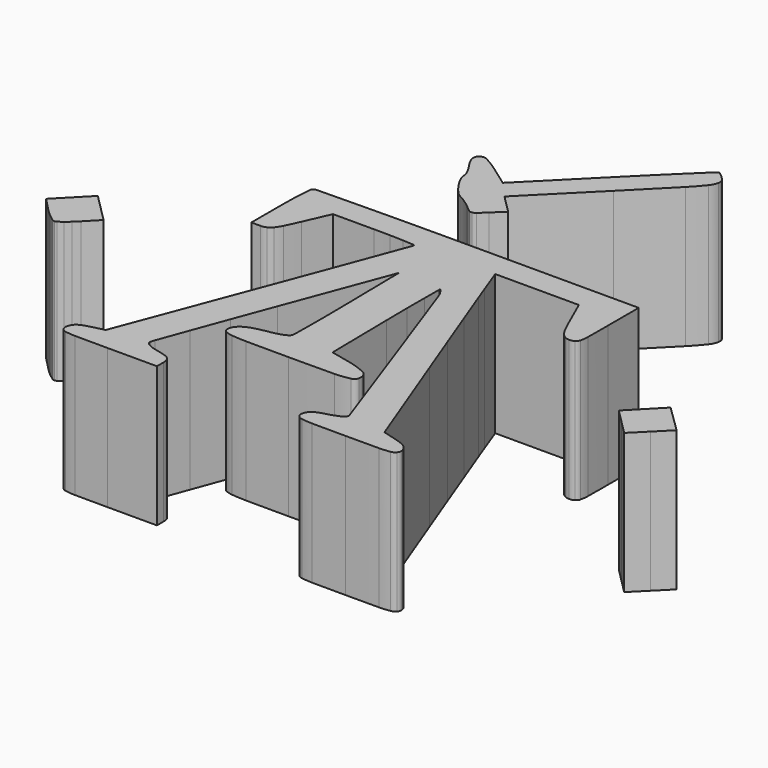
from build123d import *

# Parameters (mm, degrees)
F1_DEPTH = 25.4


# Not quite as in the source:
# - ends of sketch curves that miss each other by under 0.0002 mm in the source are joined


with BuildPart() as f1:
    # F0 (on Top) → F1 (new body)
    with BuildSketch(Plane.XY):
        with BuildLine():
            ThreePointArc((5.3278445908, 41.3714779095), (3.2465711293, 39.3070308207), (1.17245908, 37.2353889088))
            Line((1.17245908, 37.2353889088), (-9.5913702, 26.4470134))
            Line((-9.5913702, 26.4470134), (-12.7011938, 28.683204))
            ThreePointArc((-12.7011938, 28.683204), (-13.3183585785, 29.1173684963), (-13.9436757116, 29.5397069454))
            ThreePointArc((-13.9436757116, 29.5397069454), (-14.5193714679, 29.9086216736), (-15.1044112342, 30.2625312704))
            ThreePointArc((-15.1044112342, 30.2625312704), (-15.5950884738, 30.543091178), (-16.0913084379, 30.8137267723))
            ThreePointArc((-16.0913084379, 30.8137267723), (-16.2968587814, 30.8924942229), (-16.5153340201, 30.919394321))
            ThreePointArc((-16.5153340201, 30.919394321), (-16.9226686053, 30.8511854826), (-17.2859206172, 30.6546522226))
            ThreePointArc((-17.2859206172, 30.6546522226), (-17.5271690517, 30.364917692), (-17.6261968467, 30.0011334829))
            ThreePointArc((-17.6261968467, 30.0011334829), (-17.5891444827, 29.4731021199), (-17.4260613408, 28.9695197931))
            ThreePointArc((-17.4260613408, 28.9695197931), (-17.0829981706, 28.3120476284), (-16.6815115402, 27.6885323705))
            ThreePointArc((-16.6815115402, 27.6885323705), (-16.4130854245, 27.2958467266), (-16.1588952835, 26.8937997138))
            ThreePointArc((-16.1588952835, 26.8937997138), (-15.9263973461, 26.4923803768), (-15.7096472859, 26.082243352))
            ThreePointArc((-15.7096472859, 26.082243352), (-15.538374955, 25.7240460963), (-15.3811153362, 25.3594795088))
            ThreePointArc((-15.3811153362, 25.3594795088), (-15.3099545264, 25.1326203534), (-15.2773641169, 24.897105361))
            ThreePointArc((-15.2773641169, 24.897105361), (-15.1698479238, 24.2112132717), (-14.92665216, 23.5609324883))
            ThreePointArc((-14.92665216, 23.5609324883), (-14.4483979208, 22.6732535733), (-13.9104887011, 21.8204027876))
            ThreePointArc((-13.9104887011, 21.8204027876), (-13.3092790301, 21.0009126467), (-12.653090095, 20.2247464701))
            ThreePointArc((-12.653090095, 20.2247464701), (-12.116780938, 19.733761433), (-11.5001439659, 19.348471486))
            ThreePointArc((-11.5001439659, 19.348471486), (-11.1754765193, 19.1754158775), (-10.8590257516, 18.9877568523))
            ThreePointArc((-10.8590257516, 18.9877568523), (-10.478367161, 18.7427644682), (-10.1037639509, 18.488609845))
            ThreePointArc((-10.1037639509, 18.488609845), (-9.728007842, 18.2191836028), (-9.3588458321, 17.9407910626))
            ThreePointArc((-9.3588458321, 17.9407910626), (-9.0475467696, 17.6897316237), (-8.7459153929, 17.4271352824))
            ThreePointArc((-8.7459153929, 17.4271352824), (-8.3257547456, 17.0725057087), (-7.882386554, 16.7473563241))
            ThreePointArc((-7.882386554, 16.7473563241), (-7.6169836921, 16.6362047182), (-7.3292467909, 16.6373584517))
            ThreePointArc((-7.3292467909, 16.6373584517), (-7.0071387172, 16.7492612965), (-6.723922607, 16.9391689223))
            ThreePointArc((-6.723922607, 16.9391689223), (-6.0764353369, 17.5201639355), (-5.4415732409, 18.1149288306))
            Line((-5.4415732409, 18.1149288306), (-3.4675826, 20.0078086))
            Line((-3.4675826, 20.0078086), (-5.1281838, 21.6699084))
            Line((-5.1281838, 21.6699084), (-6.7888104, 23.3320082))
            Line((-6.7888104, 23.3320082), (4.1881806, 34.3331546))
            ThreePointArc((4.1881806, 34.3331546), (7.7930148251, 37.9604709487), (11.3897657807, 41.5958026114))
            ThreePointArc((11.3897657807, 41.5958026114), (12.523535317, 42.8119402167), (13.5904491586, 44.0871345239))
            ThreePointArc((13.5904491586, 44.0871345239), (14.0089149681, 44.7642866407), (14.2620308946, 45.518988275))
            ThreePointArc((14.2620308946, 45.518988275), (14.2451471296, 46.1366085958), (13.9493028376, 46.679031271))
            ThreePointArc((13.9493028376, 46.679031271), (13.705692071, 46.9401609641), (13.4545324122, 47.1940382124))
            ThreePointArc((13.4545324122, 47.1940382124), (13.2182987163, 47.4161332681), (12.9734957351, 47.6287454609))
            ThreePointArc((12.9734957351, 47.6287454609), (12.766987693, 47.794471902), (12.5548365797, 47.9529106388))
            ThreePointArc((12.5548365797, 47.9529106388), (12.4503936803, 48.0055735047), (12.3348495998, 48.0237798327))
            ThreePointArc((12.3348495998, 48.0237798327), (12.1880394684, 47.9952034702), (12.0624877712, 47.9139225334))
            ThreePointArc((12.0624877712, 47.9139225334), (10.4763017356, 46.3850143704), (8.8914892317, 44.8546824931))
            ThreePointArc((8.8914892317, 44.8546824931), (7.1047725577, 43.1180875785), (5.3278445908, 41.3714779095))
        make_face()
    extrude(amount=F1_DEPTH)


with BuildPart() as f1b:
    # F0 (on Top) → F1, piece 2 (new body)
    with BuildSketch(Plane.XY):
        with BuildLine():
            ThreePointArc((-28.9239708038, 8.2930357171), (-29.152995534, 8.2444468749), (-29.3471492398, 8.1136128535))
            ThreePointArc((-29.3471492398, 8.1136128535), (-29.4682601242, 7.9400663572), (-29.5223586626, 7.7354696381))
            ThreePointArc((-29.5223586626, 7.7354696381), (-29.5939202697, 6.8198574282), (-29.6566110746, 5.9035951827))
            ThreePointArc((-29.6566110746, 5.9035951827), (-29.7154841875, 4.8106745704), (-29.7535896341, 3.7168329073))
            ThreePointArc((-29.7535896341, 3.7168329073), (-29.7773750178, 2.4615506125), (-29.78531, 1.2060682))
            Line((-29.78531, 1.2060682), (-29.7853354, -5.26288))
            Line((-29.7853354, -5.26288), (-28.1046428, -5.26288))
            ThreePointArc((-28.1046428, -5.26288), (-27.6062777101, -5.2086551361), (-27.1310275761, -5.0491305899))
            ThreePointArc((-27.1310275761, -5.0491305899), (-26.7119543373, -4.7934727371), (-26.3618756212, -4.4493409597))
            ThreePointArc((-26.3618756212, -4.4493409597), (-25.9353004854, -3.8541164125), (-25.5779432646, -3.2149332556))
            ThreePointArc((-25.5779432646, -3.2149332556), (-24.973316268, -1.9417562352), (-24.391795328, -0.6578610928))
            Line((-24.391795328, -0.6578610928), (-22.3596454, 3.94716))
            Line((-22.3596454, 3.94716), (-14.8989034, 3.94716))
            ThreePointArc((-14.8989034, 3.94716), (-13.4684758142, 3.9410291097), (-12.0381522128, 3.922724452))
            ThreePointArc((-12.0381522128, 3.922724452), (-10.8336974413, 3.8935023943), (-9.6297757324, 3.8472710983))
            ThreePointArc((-9.6297757324, 3.8472710983), (-8.5991325983, 3.7981908828), (-7.5686922552, 3.7450220359))
            ThreePointArc((-7.5686922552, 3.7450220359), (-7.4759905736, 3.7020835845), (-7.4381868, 3.607181))
            ThreePointArc((-7.4381868, 3.607181), (-7.4503065364, 3.4718072468), (-7.4862802644, 3.3407392034))
            ThreePointArc((-7.4862802644, 3.3407392034), (-8.7724726688, -0.1083342689), (-10.0611279758, -3.5564882958))
            ThreePointArc((-10.0611279758, -3.5564882958), (-11.5008222297, -7.3994906511), (-12.9438803478, -11.2412311313))
            ThreePointArc((-12.9438803478, -11.2412311313), (-14.6549480198, -15.7720720161), (-16.3673799517, -20.3023974401))
            Line((-16.3673799517, -20.3023974401), (-25.2965712, -43.8719976))
            Line((-25.2965712, -43.8719976), (-27.7052786, -44.4677038))
            ThreePointArc((-27.7052786, -44.4677038), (-28.2874050524, -44.6307686568), (-28.8586889532, -44.8284949938))
            ThreePointArc((-28.8586889532, -44.8284949938), (-29.2562234773, -45.0160926822), (-29.6206904422, -45.261837527))
            ThreePointArc((-29.6206904422, -45.261837527), (-29.8817631628, -45.5163086696), (-30.0861395554, -45.8182124633))
            ThreePointArc((-30.0861395554, -45.8182124633), (-30.2370017448, -46.1704326022), (-30.323996421, -46.5435945421))
            ThreePointArc((-30.323996421, -46.5435945421), (-30.3007912145, -46.9830452901), (-30.1131180273, -47.3810805815))
            ThreePointArc((-30.1131180273, -47.3810805815), (-29.7883685131, -47.6800367128), (-29.375406369, -47.8359307716))
            ThreePointArc((-29.375406369, -47.8359307716), (-28.458843958, -47.95409568), (-27.5357843419, -47.99893212))
            ThreePointArc((-27.5357843419, -47.99893212), (-24.5755038228, -48.0175419738), (-21.6151714, -48.0237799114))
            Line((-21.6151714, -48.0237799114), (-12.6963424, -48.02378))
            Line((-12.6963424, -48.02378), (-12.6963424, -46.472602))
            ThreePointArc((-12.6963424, -46.472602), (-12.7302223523, -46.0551402422), (-12.8310496664, -45.6486211837))
            ThreePointArc((-12.8310496664, -45.6486211837), (-12.9862196969, -45.3438878864), (-13.2225719523, -45.0967576001))
            ThreePointArc((-13.2225719523, -45.0967576001), (-13.5940527082, -44.8590152554), (-14.0023554338, -44.6922515876))
            ThreePointArc((-14.0023554338, -44.6922515876), (-14.7423043874, -44.4823158012), (-15.4897324501, -44.3007988288))
            ThreePointArc((-15.4897324501, -44.3007988288), (-16.1129985159, -44.147980494), (-16.7292035242, -43.9688018542))
            ThreePointArc((-16.7292035242, -43.9688018542), (-17.1492723342, -43.808131553), (-17.5471652271, -43.5984765981))
            ThreePointArc((-17.5471652271, -43.5984765981), (-17.7890303402, -43.4148671659), (-17.9883130046, -43.1857457494))
            ThreePointArc((-17.9883130046, -43.1857457494), (-18.0830271411, -42.9662251402), (-18.0823332875, -42.7271440147))
            ThreePointArc((-18.0823332875, -42.7271440147), (-17.9922047416, -42.3644604005), (-17.8765595995, -42.0090894904))
            ThreePointArc((-17.8765595995, -42.0090894904), (-16.8761661379, -39.2778014924), (-15.8757102238, -36.5465363576))
            ThreePointArc((-15.8757102238, -36.5465363576), (-14.7208077115, -33.4124925221), (-13.561076035, -30.2802324757))
            ThreePointArc((-13.561076035, -30.2802324757), (-12.2081395128, -26.6521390034), (-10.8523743646, -23.025101585))
            Line((-10.8523743646, -23.025101585), (-3.823208, -4.27609))
            Line((-3.823208, -4.27609), (-3.6431474, -16.095472))
            ThreePointArc((-3.6431474, -16.095472), (-3.6136719859, -18.3874224076), (-3.5949994048, -20.6794862602))
            ThreePointArc((-3.5949994048, -20.6794862602), (-3.5906403215, -22.671554795), (-3.6006086996, -24.6636031458))
            ThreePointArc((-3.6006086996, -24.6636031458), (-3.617646112, -26.3742558468), (-3.6393185972, -28.0848561075))
            ThreePointArc((-3.6393185972, -28.0848561075), (-3.6695751202, -28.380444247), (-3.751135639, -28.6661654151))
            ThreePointArc((-3.751135639, -28.6661654151), (-3.8623048676, -28.8502564755), (-4.0302916076, -28.9845289711))
            ThreePointArc((-4.0302916076, -28.9845289711), (-4.3936920819, -29.1670538342), (-4.7676086151, -29.3269333921))
            ThreePointArc((-4.7676086151, -29.3269333921), (-5.2421745965, -29.4958060714), (-5.7260288389, -29.6358614262))
            ThreePointArc((-5.7260288389, -29.6358614262), (-6.2638999768, -29.7605658436), (-6.8069182424, -29.8605086892))
            ThreePointArc((-6.8069182424, -29.8605086892), (-8.0190343754, -30.0849752898), (-9.2190046989, -30.3672551586))
            ThreePointArc((-9.2190046989, -30.3672551586), (-10.0347957043, -30.6413342472), (-10.8059738626, -31.0233295773))
            ThreePointArc((-10.8059738626, -31.0233295773), (-11.3048691845, -31.3938263204), (-11.7115788922, -31.8636688024))
            ThreePointArc((-11.7115788922, -31.8636688024), (-11.9553040262, -32.3650301707), (-12.0390666, -32.9161648))
            ThreePointArc((-12.0390666, -32.9161648), (-11.9183040933, -33.3457718246), (-11.5913906605, -33.6495371718))
            ThreePointArc((-11.5913906605, -33.6495371718), (-10.9768409929, -33.8962944231), (-10.3275895017, -34.0268080175))
            ThreePointArc((-10.3275895017, -34.0268080175), (-8.956415452, -34.1382202475), (-7.5814175664, -34.1819462749))
            ThreePointArc((-7.5814175664, -34.1819462749), (-3.730521313, -34.202021893), (0.1204213997, -34.2087453118))
            ThreePointArc((0.1204213997, -34.2087453118), (4.2591148323, -34.1957032914), (8.3976463468, -34.1568489514))
            ThreePointArc((8.3976463468, -34.1568489514), (9.7846193058, -34.0684257366), (11.1554795133, -33.839822765))
            ThreePointArc((11.1554795133, -33.839822765), (11.6756540398, -33.5495614467), (11.9499271342, -33.0207901472))
            ThreePointArc((11.9499271342, -33.0207901472), (11.9492066699, -32.3183622866), (11.6908129953, -31.6651857299))
            ThreePointArc((11.6908129953, -31.6651857299), (11.5019501705, -31.4388791035), (11.2611464553, -31.268887852))
            ThreePointArc((11.2611464553, -31.268887852), (10.7620554787, -31.0215258697), (10.2523553101, -30.7968374028))
            ThreePointArc((10.2523553101, -30.7968374028), (9.6243180728, -30.5545425548), (8.9857341298, -30.3415904322))
            ThreePointArc((8.9857341298, -30.3415904322), (8.292834479, -30.1433250903), (7.5929489847, -29.9713396679))
            Line((7.5929489847, -29.9713396679), (4.0640254, -29.176345))
            Line((4.0640254, -29.176345), (3.8847522, -16.7660828))
            ThreePointArc((3.8847522, -16.7660828), (3.8551823479, -14.396553126), (3.8349222641, -12.0269255353))
            ThreePointArc((3.8349222641, -12.0269255353), (3.828650979, -10.0565823826), (3.835810793, -8.0862422521))
            ThreePointArc((3.835810793, -8.0862422521), (3.8489605343, -6.3857657005), (3.8644800933, -4.685309122))
            ThreePointArc((3.8644800933, -4.685309122), (3.9034557245, -4.6292112997), (3.9699407877, -4.644875361))
            ThreePointArc((3.9699407877, -4.644875361), (4.5804566767, -5.4623631608), (5.01846387, -6.3838644246))
            ThreePointArc((5.01846387, -6.3838644246), (8.2173339606, -15.3301399742), (11.410915362, -24.2783048372))
            ThreePointArc((11.410915362, -24.2783048372), (14.6850315999, -33.4763229), (17.9493538085, -42.6778213427))
            ThreePointArc((17.9493538085, -42.6778213427), (17.9716859269, -43.0784773813), (17.773638192, -43.4274853924))
            ThreePointArc((17.773638192, -43.4274853924), (17.6050453628, -43.5656397102), (17.4162550674, -43.6745783957))
            ThreePointArc((17.4162550674, -43.6745783957), (17.0602976651, -43.8353674885), (16.6993842935, -43.9847021908))
            ThreePointArc((16.6993842935, -43.9847021908), (16.2677640197, -44.1464384773), (15.8310367332, -44.2938283497))
            ThreePointArc((15.8310367332, -44.2938283497), (15.3719338033, -44.432389637), (14.9089588812, -44.5574051232))
            ThreePointArc((14.9089588812, -44.5574051232), (14.3669365543, -44.7146052049), (13.8365183342, -44.9073661764))
            ThreePointArc((13.8365183342, -44.9073661764), (13.4505758041, -45.0970991706), (13.0966666335, -45.3414319836))
            ThreePointArc((13.0966666335, -45.3414319836), (12.8387156081, -45.5939700437), (12.633215793, -45.8907599408))
            ThreePointArc((12.633215793, -45.8907599408), (12.4842625206, -46.2259033335), (12.3984867043, -46.5824838751))
            ThreePointArc((12.3984867043, -46.5824838751), (12.4272033206, -47.0131614318), (12.6302139233, -47.394073566))
            ThreePointArc((12.6302139233, -47.394073566), (12.9835009942, -47.6863609589), (13.4163811687, -47.8375498997))
            ThreePointArc((13.4163811687, -47.8375498997), (14.3847711602, -47.9542418982), (15.3591515091, -47.9987227082))
            ThreePointArc((15.3591515091, -47.9987227082), (18.4203719911, -48.0174952358), (21.4816436, -48.0237799213))
            ThreePointArc((21.4816436, -48.0237799213), (24.5291997473, -48.0174453865), (27.5767037643, -47.9985280802))
            ThreePointArc((27.5767037643, -47.9985280802), (28.5583528833, -47.9541157241), (29.5341071529, -47.8378721458))
            ThreePointArc((29.5341071529, -47.8378721458), (29.970152405, -47.6884335013), (30.3293647544, -47.3995887826))
            ThreePointArc((30.3293647544, -47.3995887826), (30.5350404946, -47.0255355391), (30.564807837, -46.5997040082))
            ThreePointArc((30.564807837, -46.5997040082), (30.4734690318, -46.2369946416), (30.3118540921, -45.8996783264))
            ThreePointArc((30.3118540921, -45.8996783264), (30.0828652781, -45.5927345053), (29.8010856701, -45.3334090197))
            ThreePointArc((29.8010856701, -45.3334090197), (29.4006427423, -45.0697274099), (28.9685803342, -44.8618681154))
            ThreePointArc((28.9685803342, -44.8618681154), (28.3527555007, -44.6348542972), (27.7256974666, -44.441018159))
            Line((27.7256974666, -44.441018159), (25.0966224, -43.7063896))
            Line((25.0966224, -43.7063896), (17.7223928, -24.3201698))
            ThreePointArc((17.7223928, -24.3201698), (16.2483975562, -20.4467436637), (14.7779953892, -16.5719521199))
            ThreePointArc((14.7779953892, -16.5719521199), (13.4021454262, -12.9487732817), (12.0298884187, -9.3242321176))
            ThreePointArc((12.0298884187, -9.3242321176), (10.8751633535, -6.2764380757), (9.7233042482, -3.2275597499))
            ThreePointArc((9.7233042482, -3.2275597499), (9.2095575325, -1.8610542829), (8.6989006445, -0.4933911882))
            Line((8.6989006445, -0.4933911882), (7.0496176, 3.94716))
            Line((7.0496176, 3.94716), (14.6317716, 3.94716))
            Line((14.6317716, 3.94716), (22.2139256, 3.94716))
            Line((22.2139256, 3.94716), (24.2461034, -0.65786))
            ThreePointArc((24.2461034, -0.65786), (24.8067119429, -1.8936261179), (25.3910406728, -3.1183546392))
            ThreePointArc((25.3910406728, -3.1183546392), (25.7561809999, -3.7756691758), (26.1862272902, -4.3924761431))
            ThreePointArc((26.1862272902, -4.3924761431), (26.5291624599, -4.7515550224), (26.9371903612, -5.0344945689))
            ThreePointArc((26.9371903612, -5.0344945689), (27.365951272, -5.2046809843), (27.8235664005, -5.2628793897))
            ThreePointArc((27.8235664005, -5.2628793897), (28.2815567719, -5.1990496136), (28.7049671228, -5.0131649933))
            ThreePointArc((28.7049671228, -5.0131649933), (29.0019809702, -4.7353184311), (29.167776369, -4.3639269133))
            ThreePointArc((29.167776369, -4.3639269133), (29.2929033693, -3.626641716), (29.3409453893, -2.8803597897))
            ThreePointArc((29.3409453893, -2.8803597897), (29.3618966899, -0.6178980304), (29.368877, 1.64465))
            Line((29.368877, 1.64465), (29.368877, 8.55218))
            Line((29.368877, 8.55218), (0.2299462, 8.55218))
            ThreePointArc((0.2299462, 8.55218), (-5.3717156885, 8.5442326998), (-10.9733332391, 8.5205792108))
            ThreePointArc((-10.9733332391, 8.5205792108), (-15.7258351947, 8.4828267231), (-20.4781148517, 8.4233411825))
            ThreePointArc((-20.4781148517, 8.4233411825), (-24.7010613421, 8.3593890045), (-28.9239708038, 8.2930357171))
        make_face()
    extrude(amount=F1_DEPTH)


with BuildPart() as f1c:
    # F0 (on Top) → F1, piece 3 (new body)
    with BuildSketch(Plane.XY):
        with BuildLine():
            Line((-51.8446766, -12.4778262), (-54.4201604, -15.1177244))
            Line((-54.4201604, -15.1177244), (-56.9956696, -17.757648))
            Line((-56.9956696, -17.757648), (-54.7637716, -20.062444))
            ThreePointArc((-54.7637716, -20.062444), (-54.316267628, -20.5104114364), (-53.8558440201, -20.9450890043))
            ThreePointArc((-53.8558440201, -20.9450890043), (-53.4219726685, -21.326212785), (-52.9736278646, -21.6901997499))
            ThreePointArc((-52.9736278646, -21.6901997499), (-52.5952995616, -21.9739214212), (-52.2074018123, -22.2444128626))
            ThreePointArc((-52.2074018123, -22.2444128626), (-52.0147287362, -22.3357607457), (-51.8038333997, -22.3672396999))
            ThreePointArc((-51.8038333997, -22.3672396999), (-51.5927363619, -22.3356797222), (-51.399933274, -22.2441102888))
            ThreePointArc((-51.399933274, -22.2441102888), (-51.0106739311, -21.97217251), (-50.6309764169, -21.6870361582))
            ThreePointArc((-50.6309764169, -21.6870361582), (-50.1809380234, -21.3213231305), (-49.7453971475, -20.938458968))
            ThreePointArc((-49.7453971475, -20.938458968), (-49.2829708641, -20.5017055521), (-48.8334660596, -20.0516644471))
            Line((-48.8334660596, -20.0516644471), (-46.5911438, -17.7360834))
            Line((-46.5911438, -17.7360834), (-49.2179102, -15.1069548))
            Line((-49.2179102, -15.1069548), (-51.8446766, -12.4778262))
        make_face()
    extrude(amount=F1_DEPTH)


with BuildPart() as f1d:
    # F0 (on Top) → F1, piece 4 (new body)
    with BuildSketch(Plane.XY):
        Polygon((51.985926, -12.4961396), (49.4072672, -15.139289), (46.8286084, -17.7824638), (49.272952, -20.2289918), (51.7172956, -22.6755452), (54.3564826, -20.0339706), (56.9956696, -17.3924214), (54.4907978, -14.9442678), align=None)
    extrude(amount=F1_DEPTH)


solid = Compound([f1.part, f1b.part, f1c.part, f1d.part])
